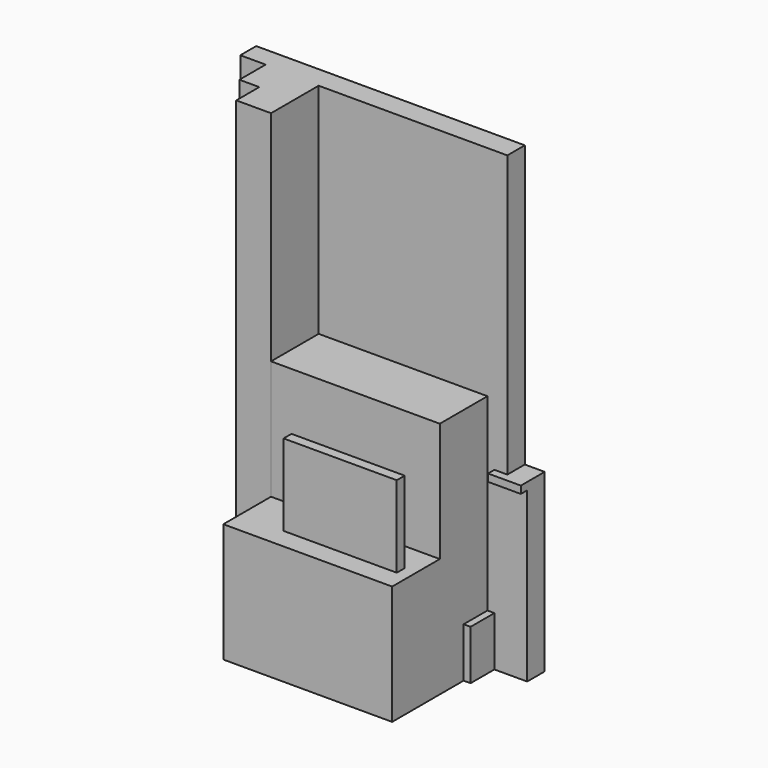
from build123d import *

# Parameters (mm, degrees)
F0_W     = 10
F0_H     = 11
F1_DEPTH = 88.5
F2_START = 84.8
F2_DEPTH = 3.7
F3_DEPTH = 230
F4_DEPTH = 25
F5_W     = 85
F5_H     = 30
F6_DEPTH = 60
F7_DEPTH = 120
F8_W     = 57
F8_H     = 5
F9_DEPTH = 41


with BuildPart() as f1:
    # F0 (on Top) → F1 (new body)
    with BuildSketch(Plane.XY):
        Polygon((0, -15), (0, 0), (88.5, 0), (95, 0), (95, 11), (-40.2532453754, 11), (-40.2532453754, 1), (-27.5, 1), (-27.5, -15.5), (-17.5, -15.5), (-17.5, -30), (0, -30), align=None)
        with Locations((100, 5.5)):
            Rectangle(F0_W, F0_H)
    extrude(amount=F1_DEPTH)

    # F0 (on Top) → F2 (join)
    with BuildSketch(Plane.XY.offset(F2_START)):
        Polygon((95, 0), (88.5, 0), (88.5, -4), (105, -4), (105, 0), align=None)
    extrude(amount=F2_DEPTH)

    # F0 (on Top) → F3 (join)
    with BuildSketch(Plane.XY):
        Polygon((0, -15), (0, 0), (88.5, 0), (95, 0), (95, 11), (-40.2532453754, 11), (-40.2532453754, 1), (-27.5, 1), (-27.5, -15.5), (-17.5, -15.5), (-17.5, -30), (0, -30), align=None)
    extrude(amount=F3_DEPTH)

    # F0 (on Top) → F4 (join)
    with BuildSketch(Plane.XY):
        Polygon((88.5, 0), (0, 0), (0, -15), (88.5, -15), (88.5, -4), align=None)
    extrude(amount=F4_DEPTH)


with BuildPart() as f6:
    # F5 (on Top) → F6 (new body)
    with BuildSketch(Plane.XY):
        with Locations((42.5, -15)):
            Rectangle(F5_W, F5_H)
        with Locations((42.5, -45)):
            Rectangle(F5_W, F5_H)
    extrude(amount=F6_DEPTH)

    # F5 (on Top) → F7 (join)
    with BuildSketch(Plane.XY):
        with Locations((42.5, -15)):
            Rectangle(F5_W, F5_H)
    extrude(amount=F7_DEPTH)


with BuildPart() as f9:
    # F8 (on face) → F9 (new body)
    with BuildSketch(Plane.XY.offset(60)):
        with Locations((50.5448982381, -47.157112509)):
            Rectangle(F8_W, F8_H)
    extrude(amount=F9_DEPTH)


solid = Compound([f1.part, f6.part, f9.part])
